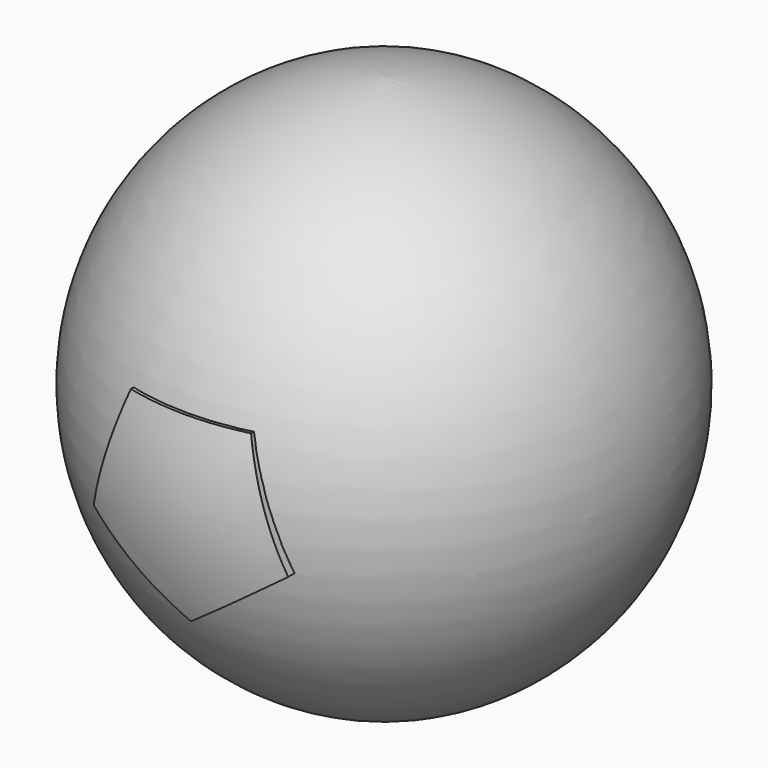
from build123d import *

# Parameters (mm, degrees)
F4_DEPTH = 25.4


with BuildPart() as f1:
    # F0 (on Front) → F1 (revolve)
    with BuildSketch(Plane.XZ):
        with BuildLine():
            ThreePointArc((0, -25.1227747649), (24.5493442784, 0.8185785264), (0, 26.7599318177))
            Line((0, 26.7599318177), (0, -25.1227747649))
        make_face()
    revolve(axis=Axis((0, 0, 0.8185785264), (0, 0, -1)))


with BuildPart() as f4:
    # F3 (on offset) → F4 (new body)
    with BuildSketch(Plane.XZ.offset(25.4)):
        Polygon((5.766931316, 7.9375), (-5.766931316, 7.9375), (-9.3310908801, -3.0318552143), (0, -9.8112895714), (9.3310908801, -3.0318552143), align=None)
    extrude(amount=-F4_DEPTH)

    # F5 (on Top) → F6 (revolve, cut)
    with BuildSketch(Plane.XY):
        with BuildLine():
            ThreePointArc((25.146, 0), (17.7809071197, -17.7809071197), (0, -25.146))
            Line((0, -25.146), (0, -31.1810316509))
            Line((0, -31.1810316509), (30.6788852322, -31.1810316509))
            Line((30.6788852322, -31.1810316509), (30.6788852322, 0))
            Line((30.6788852322, 0), (25.146, 0))
        make_face()
    revolve(axis=Axis((0, -12.573, 0), (0, -1, 0)), mode=Mode.SUBTRACT)


solid = Compound([f1.part, f4.part])
